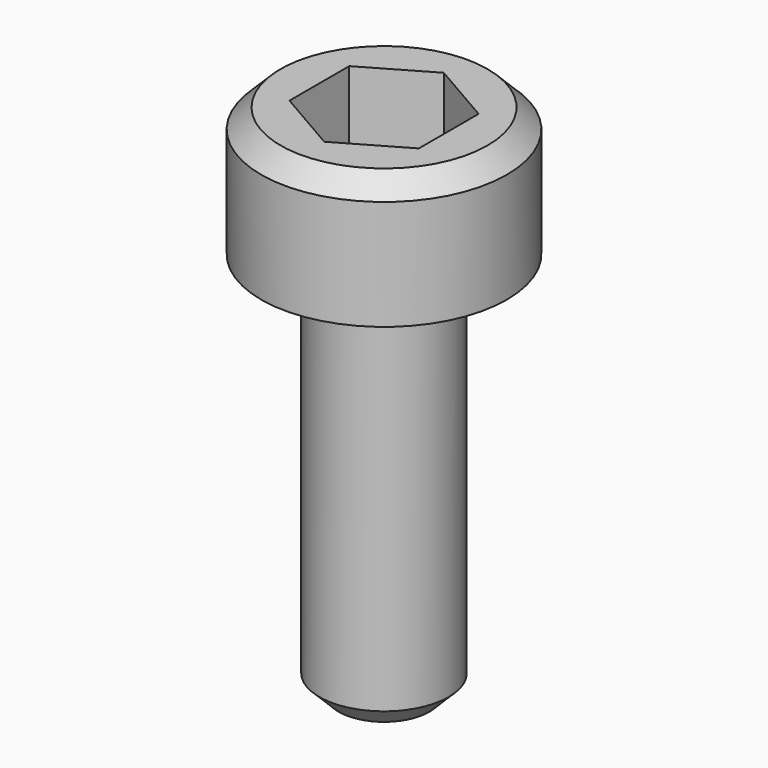
from build123d import *

# Parameters (mm, degrees)
F2_R      = 1
F3_DEPTH  = 6
F2_R_2    = 1.9
F3_FACE_R = 1
F4_DEPTH  = 2
F5_SIZE   = 0.3
F7_DEPTH  = 1.3


with BuildPart() as f3:
    # F2 (on Top) → F3 (new body)
    with BuildSketch(Plane.XY):
        Circle(F2_R)
    extrude(amount=-F3_DEPTH)

    # F2 (on Top) + F3_face (on face) → F4 (join)
    with BuildSketch(Plane.XY):
        Circle(F2_R_2)
        Circle(F2_R, mode=Mode.SUBTRACT)
    with BuildSketch(Plane.XY):
        Circle(F3_FACE_R)
    extrude(amount=F4_DEPTH)

    # F5
    f5_edges = [f3.edges().sort_by_distance(p)[0] for p in [
        (-1, 0, -6),
        (-1.9, 0, 2),
    ]]
    chamfer(f5_edges, length=F5_SIZE)

    # F6 (on face) → F7 (cut)
    with BuildSketch(Plane.XY.offset(2)):
        Polygon((1, -0.5773502692), (1, 0.5773502692), (0, 1.1547005384), (-1, 0.5773502692), (-1, -0.5773502692), (0, -1.1547005384), align=None)
    extrude(amount=-F7_DEPTH, mode=Mode.SUBTRACT)


solid = f3.part
